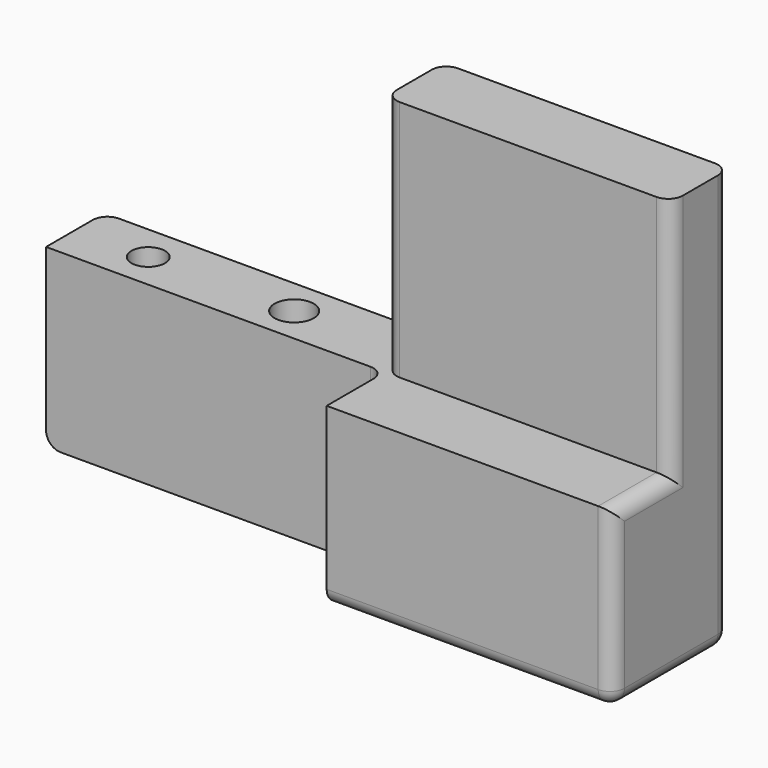
from build123d import *

# Parameters (mm, degrees)
F1_DEPTH    = 25.4
F2_R        = 5.8227150046
F2_R_2      = 6.8159523424
F3_DEPTH    = 152.4
F4_W        = 99.5925068855
F4_H        = 61.3070130348
F5_DEPTH    = 25.4
F6_T1_DEPTH = 61.3070130348
F7_R        = 5.08
F8_R        = 5.08
F9_R        = 5.08
F10_R       = 5.08
F11_R       = 5.08
F12_R       = 5.08
F13_R       = 5.08


# Not quite as in the source:
# - a fillet or chamfer that OpenCascade refuses, or shapes differently, is made with other operations: its cross-section is extruded or revolved along the edge and cut away or added


with BuildPart() as f1:
    # F0 (on Front) → F1 (new body)
    with BuildSketch(Plane.XZ):
        Polygon((118.0045455694, 0), (0, 0), (0, -61.3070130348), (217.5970524549, -61.3070130348), (217.5970524549, 84.4091549516), (118.0045455694, 84.4091549516), align=None)
    extrude(amount=F1_DEPTH)

    # F2 (on face) → F3 (cut)
    with BuildSketch(Plane.XY):
        with Locations((25.4, -12.7)):
            Circle(F2_R)
        with Locations((76.2, -12.7)):
            Circle(F2_R_2)
    extrude(amount=-F3_DEPTH, mode=Mode.SUBTRACT)

    # F4 (on face) → F5 (join)
    with BuildSketch(Plane.XZ.offset(25.4)):
        with Locations((167.8007990122, -30.6535065174)):
            Rectangle(F4_W, F4_H)
    extrude(amount=F5_DEPTH)

    # F6: fillet of radius 5.08 on 1 edges, made by hand

    # F6_s2 → F6_t1 (join)
    with BuildSketch(Plane.XY.offset(-61.3070130348)):
        with BuildLine():
            ThreePointArc((118.0045455694, -30.48), (116.5166480178, -26.8878975516), (112.9245455694, -25.4))
            Line((112.9245455694, -25.4), (118.0045455694, -25.4))
            Line((118.0045455694, -25.4), (118.0045455694, -30.48))
        make_face()
    extrude(amount=F6_T1_DEPTH)

    # F7
    f7_edges = [f1.edges().sort_by_distance(p)[0] for p in [
        (118.004546, -25.4, 42.204577),
    ]]
    fillet(f7_edges, radius=F7_R)

    # F8
    f8_edges = [f1.edges().sort_by_distance(p)[0] for p in [
        (217.597052, -25.4, 42.204577),
    ]]
    fillet(f8_edges, radius=F8_R)

    # F9
    f9_edges = [f1.edges().sort_by_distance(p)[0] for p in [
        (217.597052, -38.1, 0),
        (217.597052, -50.8, -30.653507),
    ]]
    fillet(f9_edges, radius=F9_R)

    # F10
    f10_edges = [f1.edges().sort_by_distance(p)[0] for p in [
        (217.597052, -22.86, -61.307013),
    ]]
    fillet(f10_edges, radius=F10_R)

    # F11
    f11_edges = [f1.edges().sort_by_distance(p)[0] for p in [
        (217.597052, 0, 14.091071),
    ]]
    fillet(f11_edges, radius=F11_R)

    # F12
    f12_edges = [f1.edges().sort_by_distance(p)[0] for p in [
        (118.004546, 0, 42.204577),
    ]]
    fillet(f12_edges, radius=F12_R)

    # F13
    f13_edges = [f1.edges().sort_by_distance(p)[0] for p in [
        (0, 0, -28.113507),
        (0, -1.487898, -59.819115),
        (0, -15.24, -61.307013),
    ]]
    fillet(f13_edges, radius=F13_R)


solid = f1.part
